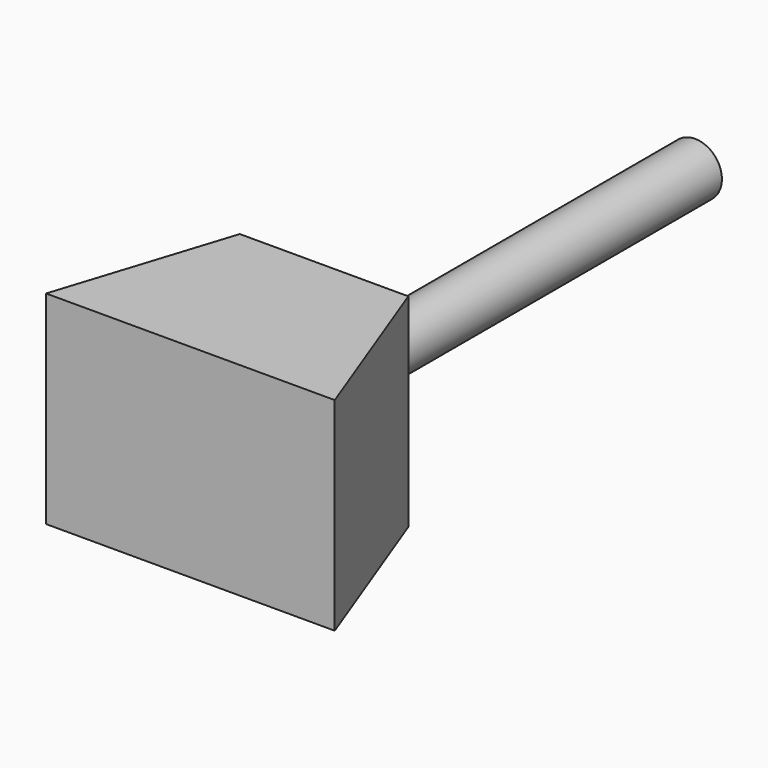
from build123d import *

# Parameters (mm, degrees)
F1_DEPTH = 25.4
F2_DEPTH = 50.8
F3_R     = 10.0458196752
F4_DEPTH = 203.2


# Not quite as in the source:
# - the program builds the solid bodies; features that only make, move or delete a surface that nothing else refers to are left out


with BuildPart() as f1:
    # F0 (on Top) → F1 (new body)
    with BuildSketch(Plane.XY):
        Polygon((28.6761522293, 32.8064598143), (-34.5765948296, 32.8064598143), (-55.3461499512, -32.0984050632), (52.9859773815, -32.0984050632), align=None)
    extrude(amount=F1_DEPTH)

    # F2 (add): a face of the model
    f2_faces = [f1.faces().sort_by_distance(p)[0] for p in [
        (-1.9876444454, -2.4879782653, 0),
    ]]
    extrude(f2_faces, amount=F2_DEPTH)

    # F3 (on Front) → F4 (join)
    with BuildSketch(Plane.XZ):
        with Locations((0, -11.2053733319)):
            Circle(F3_R)
    extrude(amount=-F4_DEPTH)


solid = f1.part
